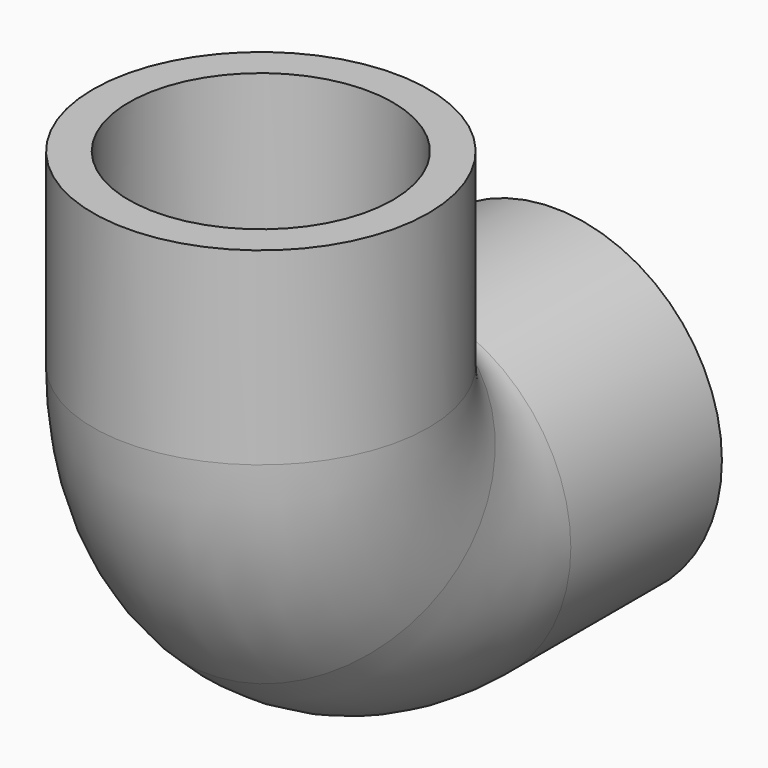
from build123d import *
from build123d import SkipClean  # not in build123d's __all__

# Parameters (mm, degrees)
F0_R        = 16.7005
F0_R_2      = 13.1191
F1_DEPTH    = 2.54
F0_R_3      = 21.209
F2_DEPTH    = 23.876
F2_FACE_R   = 21.209
F2_FACE_R_2 = 13.1191
F5_ANGLE    = 45


with BuildPart() as f1:
    # F0 (on Top) → F1 (new body)
    with BuildSketch(Plane.XY):
        Circle(F0_R)
        Circle(F0_R_2, mode=Mode.SUBTRACT)
    extrude(amount=F1_DEPTH)

    # F0 (on Top) → F2 (join)
    with BuildSketch(Plane.XY):
        Circle(F0_R_3)
        Circle(F0_R, mode=Mode.SUBTRACT)
    extrude(amount=F2_DEPTH)

    # F2_face (on face) → F5 (revolve)
    with BuildSketch(Plane(origin=(0, 0, 0), x_dir=(1, 0, 0), z_dir=(0, 0, -1))):
        Circle(F2_FACE_R)
        Circle(F2_FACE_R_2, mode=Mode.SUBTRACT)
    revolve(axis=Axis((12.7, 22.479, 0), (1, 0, 0)), revolution_arc=F5_ANGLE)

    # F6: F1 across face


with BuildPart() as f1_1:
    add(f1.part, clean=False)
    with SkipClean():  # cleaning this boolean's faces spoils the solid; the shape is the same uncleaned
        add(f1.part.mirror(Plane(origin=(0, 6.5839466657, -15.8950533343), x_dir=(-1, 0, 0), z_dir=(0, 0.7071067812, -0.7071067812))), clean=False)


solid = f1_1.part
